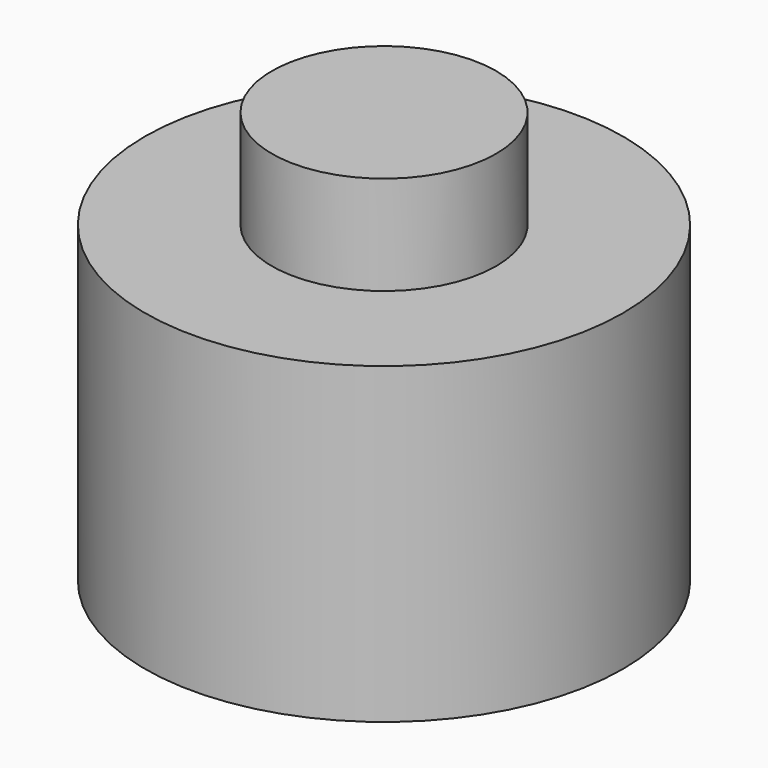
from build123d import *

# Parameters (mm, degrees)
F0_R     = 14.5
F1_DEPTH = 19
F2_R     = 6.8
F3_DEPTH = 6
F4_W     = 10.5
F4_H     = 10.5
F5_DEPTH = 10


# Not quite as in the source:
# - a feature of the source that left no trace in its solid (it failed there, or was rolled back) is left out


with BuildPart() as f1:
    # F0 (on Top) → F1 (new body)
    with BuildSketch(Plane.XY):
        Circle(F0_R)
    extrude(amount=F1_DEPTH)

    # F2 (on face) → F3 (join)
    with BuildSketch(Plane.XY.offset(19)):
        Circle(F2_R)
    extrude(amount=F3_DEPTH)

    # F4 (on face) → F5 (cut)
    with BuildSketch(Plane(origin=(0, 0, 0), x_dir=(1, 0, 0), z_dir=(0, 0, -1))):
        Rectangle(F4_W, F4_H)
    extrude(amount=-F5_DEPTH, mode=Mode.SUBTRACT)


solid = f1.part
